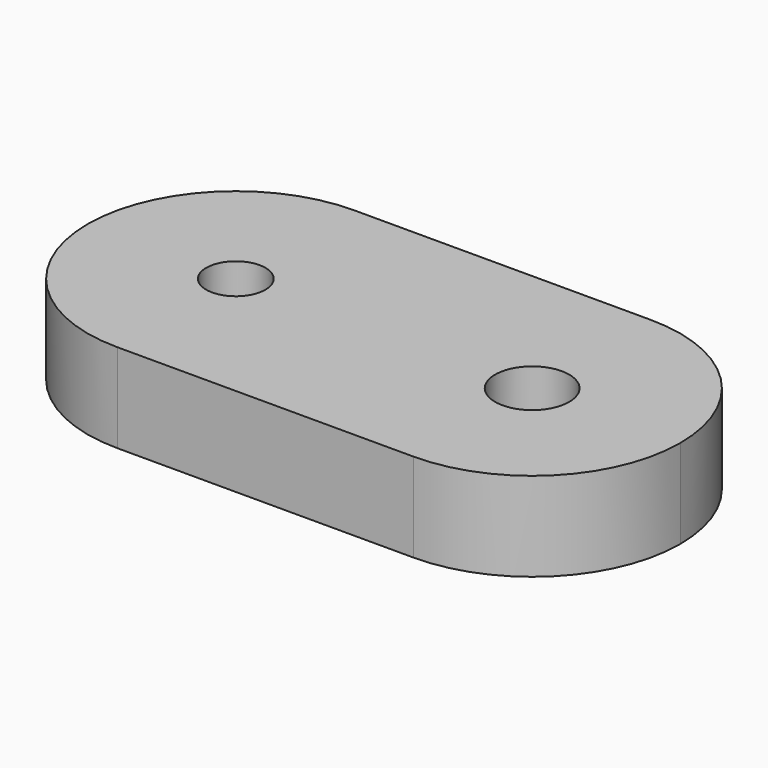
from build123d import *

# Parameters (mm, degrees)
F0_R     = 2.5
F0_R_2   = 2
F1_DEPTH = 6
F2_DEPTH = 3.2
F3_R     = 9.99999


# Not quite as in the source:
# - a fillet or chamfer is up to 0.001 mm smaller than in the source, because OpenCascade refuses the exact size


with BuildPart() as f1:
    # F0 (on Top) → F1 (new body)
    with BuildSketch(Plane.XY):
        Polygon((20, -10), (20, 10), (0, 10), (-20, 10), (-20, -10), (0, -10), align=None)
        Polygon((-10, 4.0414518843), (-6.5, 2.0207259422), (-6.5, -2.0207259422), (-10, -4.0414518843), (-13.5, -2.0207259422), (-13.5, 2.0207259422), align=None, mode=Mode.SUBTRACT)
        with Locations((10, 0)):
            Circle(F0_R, mode=Mode.SUBTRACT)
        Polygon((-6.5, -2.0207259422), (-6.5, 2.0207259422), (-10, 4.0414518843), (-13.5, 2.0207259422), (-13.5, -2.0207259422), (-10, -4.0414518843), align=None)
        with Locations((-10, 0)):
            Circle(F0_R_2, mode=Mode.SUBTRACT)
    extrude(amount=F1_DEPTH)

    # F0 (on Top) → F2 (cut)
    with BuildSketch(Plane.XY):
        Polygon((-6.5, -2.0207259422), (-6.5, 2.0207259422), (-10, 4.0414518843), (-13.5, 2.0207259422), (-13.5, -2.0207259422), (-10, -4.0414518843), align=None)
        with Locations((-10, 0)):
            Circle(F0_R_2, mode=Mode.SUBTRACT)
    extrude(amount=F2_DEPTH, mode=Mode.SUBTRACT)

    # F3 (radius 10 in the source; OpenCascade refuses exactly that, so slightly less here)
    f3_edges = [f1.edges().sort_by_distance(p)[0] for p in [
        (-20, -10, 3),
        (20, -10, 3),
        (20, 10, 3),
        (-20, 10, 3),
    ]]
    fillet(f3_edges, radius=F3_R)


solid = f1.part
